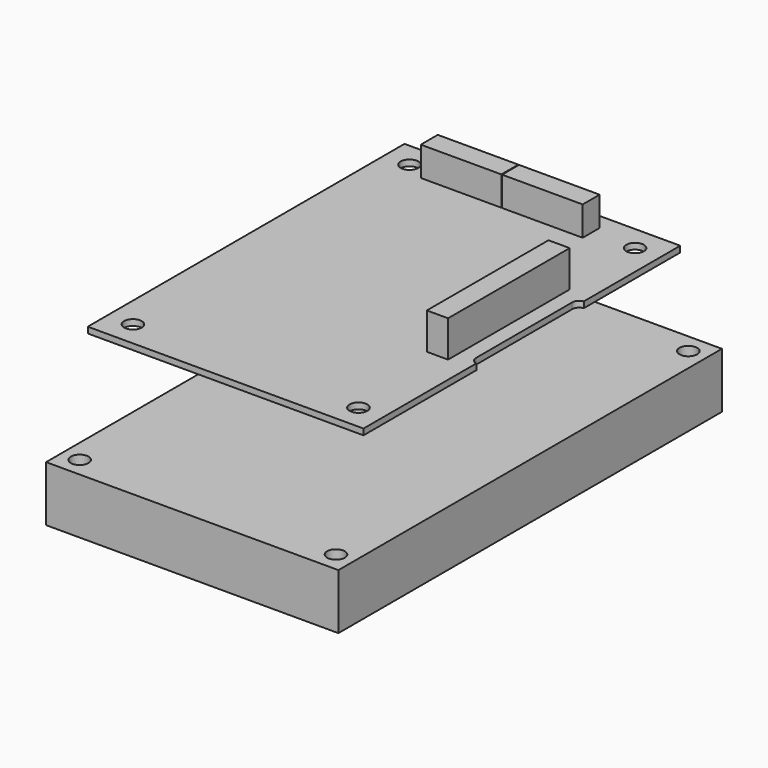
from build123d import *

# Parameters (mm, degrees)
F0_W         = 41.35
F0_H         = 67.8
F1_DEPTH     = 7.85
F2_R         = 1.25
F3_DEPTH     = 7.851
F5_W         = 39
F5_H         = 56
F6_DEPTH     = 0.85
F7_R         = 1.25
F8_DEPTH     = 22.701
F9_W         = 3
F9_H         = 21.5
F10_DEPTH    = 5.15
F9_W_2       = 11.4
F9_H_2       = 3
F11_DEPTH    = 4.15
F12_W        = 0.85
F12_H        = 19
F13_DEPTH    = 22.701
F14_T1_DEPTH = 0.85


# Not quite as in the source:
# - a fillet or chamfer that OpenCascade refuses, or shapes differently, is made with other operations: its cross-section is extruded or revolved along the edge and cut away or added


with BuildPart() as f1:
    # F0 (on Top) → F1 (new body)
    with BuildSketch(Plane.XY):
        Rectangle(F0_W, F0_H)
    extrude(amount=F1_DEPTH)

    # F2 (on face) → F3 (cut, through all)
    with BuildSketch(Plane.XY.offset(7.85)):
        with Locations((-18.125, -31.15)):
            Circle(F2_R)
        with Locations((-18.125, 31.15)):
            Circle(F2_R)
        with Locations((18.125, 31.15)):
            Circle(F2_R)
        with Locations((18.125, -31.15)):
            Circle(F2_R)
    extrude(amount=-F3_DEPTH, mode=Mode.SUBTRACT)


with BuildPart() as f6:
    # F5 (on offset) → F6 (new body)
    with BuildSketch(Plane.XY.offset(21.85)):
        Rectangle(F5_W, F5_H)
    extrude(amount=F6_DEPTH)

    # F7 (on face) → F8 (cut, through all)
    with BuildSketch(Plane.XY.offset(22.7)):
        with Locations((-15.95, 24.45)):
            Circle(F7_R)
        with Locations((-15.95, -24.45)):
            Circle(F7_R)
        with Locations((15.95, 24.45)):
            Circle(F7_R)
        with Locations((15.95, -24.45)):
            Circle(F7_R)
    extrude(amount=-F8_DEPTH, mode=Mode.SUBTRACT)

    # F12 (on face) → F13 (cut, through all)
    with BuildSketch(Plane.XY.offset(22.7)):
        with Locations((19.075, 1.45)):
            Rectangle(F12_W, F12_H)
    extrude(amount=-F13_DEPTH, mode=Mode.SUBTRACT)

    # F14: fillet of radius 1 on 2 edges, made by hand

    # F14_s2 → F14_t1 (join)
    with BuildSketch(Plane.XY.offset(21.85)):
        with BuildLine():
            ThreePointArc((19.5, 10.95), (18.8917124556, 10.6132342439), (18.65, 9.9613140033))
            Line((18.65, 9.9613140033), (18.65, 10.95))
            Line((18.65, 10.95), (19.5, 10.95))
        make_face()
        with BuildLine():
            ThreePointArc((18.65, -7.0613140033), (18.8917124556, -7.7132342439), (19.5, -8.05))
            Line((19.5, -8.05), (18.65, -8.05))
            Line((18.65, -8.05), (18.65, -7.0613140033))
        make_face()
    extrude(amount=F14_T1_DEPTH)


with BuildPart() as f10:
    # F9 (on face) → F10 (new body)
    with BuildSketch(Plane.XY.offset(22.7)):
        with Locations((15, 1.45)):
            Rectangle(F9_W, F9_H)
    extrude(amount=F10_DEPTH)


with BuildPart() as f11:
    # F9 (on face) → F11 (new body)
    with BuildSketch(Plane.XY.offset(22.7)):
        with Locations((-7.3, 24.25)):
            Rectangle(F9_W_2, F9_H_2)
    extrude(amount=F11_DEPTH)


with BuildPart() as f11b:
    # F9 (on face) → F11, piece 2 (new body)
    with BuildSketch(Plane.XY.offset(22.7)):
        with Locations((4.2, 24.25)):
            Rectangle(F9_W_2, F9_H_2)
    extrude(amount=F11_DEPTH)


solid = Compound([f1.part, f6.part, f10.part, f11.part, f11b.part])
